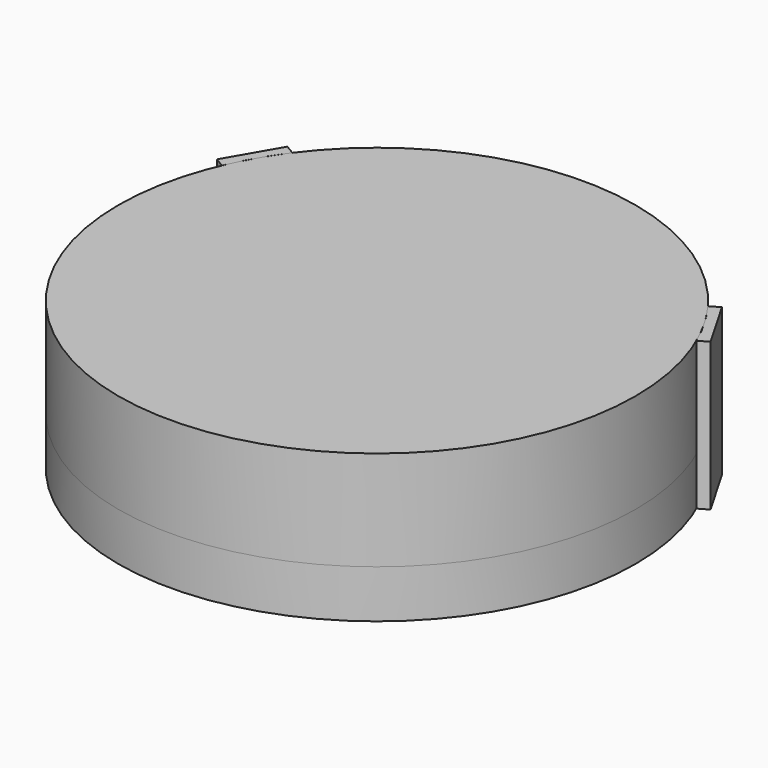
from build123d import *

# Parameters (mm, degrees)
F0_R      = 3500
F1_DEPTH  = 1350
F7_DEPTH  = 2000
F9_R      = 3500
F10_DEPTH = 650


# Not quite as in the source:
# - the program builds the solid bodies; features that only make, move or delete a surface that nothing else refers to are left out


with BuildPart() as f1:
    # F0 (on Top) → F1 (new body)
    with BuildSketch(Plane.XY):
        Circle(F0_R)
    extrude(amount=F1_DEPTH)


with BuildPart() as f7:
    # F6 (on face) → F7 (new body)
    with BuildSketch(Plane.XY.offset(1350)):
        with BuildLine():
            Line((-3341.1327955504, 1467.1237035576), (-3211.2289849827, 1392.1237035576))
            ThreePointArc((-3211.2289849827, 1392.1237035576), (-3126.2840636327, 1573.6416216776), (-3031.0889132455, 1750))
            Line((-3031.0889132455, 1750), (-3141.1327955504, 1813.5338650714))
            Line((-3141.1327955504, 1813.5338650714), (-3341.1327955504, 1467.1237035576))
        make_face()
        with BuildLine():
            Line((-3141.1327955504, 1813.5338650714), (-3031.0889132455, 1750))
            ThreePointArc((-3031.0889132455, 1750), (-2925.9556526417, 1920.6206077136), (-2811.2289849827, 2084.9440265851))
            Line((-2811.2289849827, 2084.9440265851), (-2941.1327955504, 2159.9440265851))
            Line((-2941.1327955504, 2159.9440265851), (-3141.1327955504, 1813.5338650714))
        make_face()
    extrude(amount=-F7_DEPTH)


with BuildPart() as f7b:
    # F6 (on face) → F7, piece 2 (new body)
    with BuildSketch(Plane.XY.offset(1350)):
        with BuildLine():
            ThreePointArc((2811.2289849827, 2084.9440265851), (2925.9556526417, 1920.6206077136), (3031.0889132455, 1750))
            Line((3031.0889132455, 1750), (3141.1327955504, 1813.5338650714))
            Line((3141.1327955504, 1813.5338650714), (2941.1327955504, 2159.9440265851))
            Line((2941.1327955504, 2159.9440265851), (2811.2289849827, 2084.9440265851))
        make_face()
        with BuildLine():
            ThreePointArc((3031.0889132455, 1750), (3126.2840636327, 1573.6416216776), (3211.2289849827, 1392.1237035576))
            Line((3211.2289849827, 1392.1237035576), (3341.1327955504, 1467.1237035576))
            Line((3341.1327955504, 1467.1237035576), (3141.1327955504, 1813.5338650714))
            Line((3141.1327955504, 1813.5338650714), (3031.0889132455, 1750))
        make_face()
    extrude(amount=-F7_DEPTH)


with BuildPart() as f10:
    # F9 (on offset) → F10 (new body)
    with BuildSketch(Plane(origin=(0, 0, 0), x_dir=(1, 0, 0), z_dir=(0, 0, -1))):
        Circle(F9_R)
    extrude(amount=F10_DEPTH)


solid = Compound([f1.part, f7.part, f7b.part, f10.part])
